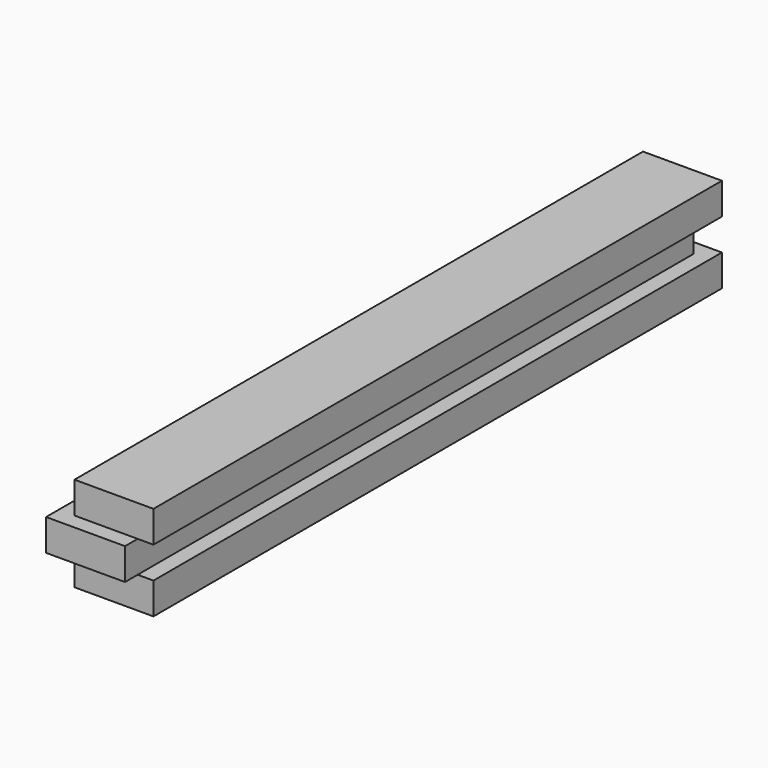
from build123d import *

# Parameters (mm, degrees)
F2_W     = 7.9375
F2_H     = 71.4375
F3_DEPTH = 3.175
F4_W     = 7.9375
F4_H     = 71.4375
F5_DEPTH = 3.175
F6_W     = 7.9375
F6_H     = 71.4375
F7_DEPTH = 3.175


# Not quite as in the source:
# - a variable given as a bare number and used for a length is read in inches; the dataset says mm whatever the document's units were


with BuildPart() as f3:
    # F2 (on Top) → F3 (new body)
    with BuildSketch(Plane.XY):
        with Locations((3.96875, 35.71875)):
            Rectangle(F2_W, F2_H)
    extrude(amount=F3_DEPTH)

    # F4 (on face) → F5 (join)
    with BuildSketch(Plane.XY.offset(3.175)):
        with Locations((2.38125, 34.13125)):
            Rectangle(F4_W, F4_H)
    extrude(amount=F5_DEPTH)

    # F6 (on face) → F7 (join)
    with BuildSketch(Plane.XY.offset(6.35)):
        with Locations((3.96875, 35.71875)):
            Rectangle(F6_W, F6_H)
    extrude(amount=F7_DEPTH)


solid = f3.part
